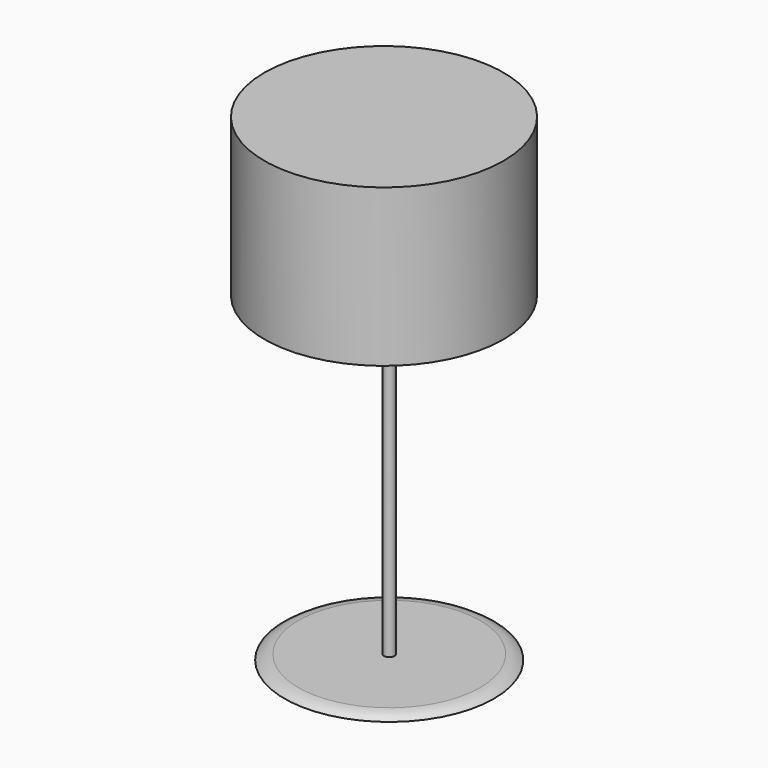
from build123d import *

# Parameters (mm, degrees)
F0_R     = 25.4
F1_DEPTH = 1.27
F3_R     = 1.27
F4_DEPTH = 76.2
F5_R     = 28.9937476924
F6_DEPTH = 38.1


# Not quite as in the source:
# - a fillet or chamfer that OpenCascade refuses, or shapes differently, is made with other operations: its cross-section is extruded or revolved along the edge and cut away or added


with BuildPart() as f1:
    # F0 (on Top) → F1 (new body)
    with BuildSketch(Plane.XY):
        Circle(F0_R)
    extrude(amount=F1_DEPTH)

    # F2: fillet of radius 5.08 on 1 edges, made by hand

    # F2_s1 → F2_t2 (revolve, cut)
    with BuildSketch(Plane.XZ):
        with BuildLine():
            ThreePointArc((25.4, 0), (23.8359470592, 0.9419048812), (22.0398958349, 1.27))
            Line((22.0398958349, 1.27), (25.4, 1.27))
            Line((25.4, 1.27), (25.4, 0))
        make_face()
    revolve(axis=Axis((0, 0, 1.27), (0, 0, 1)), mode=Mode.SUBTRACT)

    # F3 (on face) → F4 (join)
    with BuildSketch(Plane.XY.offset(1.27)):
        Circle(F3_R)
    extrude(amount=F4_DEPTH)

    # F5 (on face) → F6 (join)
    with BuildSketch(Plane.XY.offset(77.47)):
        with Locations((-1.27, 0)):
            Circle(F5_R)
    extrude(amount=F6_DEPTH)


solid = f1.part
